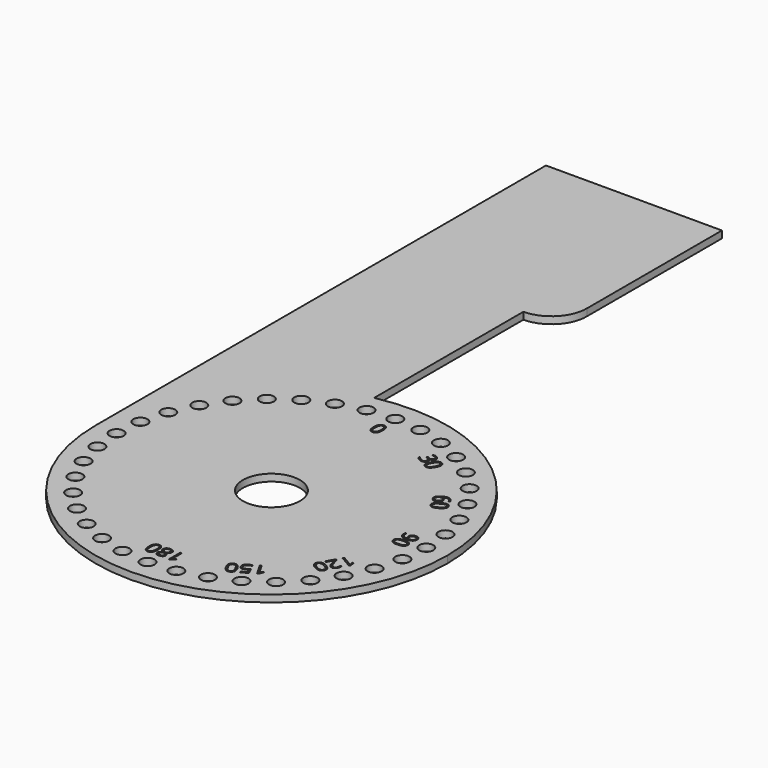
from build123d import *

# Parameters (mm, degrees)
F1_DEPTH     = 1
F3_D         = 2
F4_TEXT_SIZE = 2.7777777778
F5_DEPTH     = 1
F6_TEXT_SIZE = 2.7777777778
F7_DEPTH     = 25
F8_TEXT_SIZE = 2.7777777778
F9_DEPTH     = 25
F11_DEPTH    = 1


# Not quite as in the source:
# - a feature names something its author has since deleted; it is built from what else it names
# - Text() gives the source's letters only with a copy of the font that has no kerning and outlines rounded to 1/6400 em; it was checked with that copy


with BuildPart() as f1:
    # F0 (on Top) → F1 (new body)
    with BuildSketch(Plane.XY):
        with BuildLine():
            ThreePointArc((-25, 0), (0, 25), (25, 0))
            Line((25, 0), (25, 35))
            Line((25, 35), (0, 60))
            Line((0, 60), (0, 65))
            Line((0, 65), (25, 65))
            Line((25, 65), (25, 80))
            Line((25, 80), (-25, 80))
            Line((-25, 80), (-25, 0))
        make_face()
        with BuildLine():
            Line((25, 0), (4.05, 0))
            ThreePointArc((4.05, 0), (0, -4.05), (-4.05, 0))
            Line((-4.05, 0), (-25, 0))
            ThreePointArc((-25, 0), (0, -25), (25, 0))
        make_face()
        with BuildLine():
            ThreePointArc((-4.05, 0), (0, 4.05), (4.05, 0))
            Line((4.05, 0), (25, 0))
            ThreePointArc((25, 0), (0, 25), (-25, 0))
            Line((-25, 0), (-4.05, 0))
        make_face()
        Polygon((0, 60), (25, 35), (25, 65), (0, 65), align=None)
    extrude(amount=-F1_DEPTH)

    # F3 (through all)
    with Locations(Plane.XY):
        with Locations((0, -22), (0, 0), (7.5244431532, -20.6732376573), (3.8202599087, -21.6657705663), (-22, 0), (21.6657705663, -3.8202599087), (-21.6657705663, -3.8202599087), (19.0525588833, -11), (-16.8529777486, 14.1413274131), (-21.6657705663, 3.8202599087), (16.8529777486, 14.1413274131), (-7.5244431532, -20.6732376573), (-7.5244431532, 20.6732376573), (-14.1413274131, 16.8529777486), (22, 0), (-14.1413274131, -16.8529777486), (-20.6732376573, 7.5244431532), (-16.8529777486, -14.1413274131), (14.1413274131, -16.8529777486), (11, 19.0525588833), (-19.0525588833, 11), (-20.6732376573, -7.5244431532), (20.6732376573, -7.5244431532), (3.8202599087, 21.6657705663), (0, 22), (-11, -19.0525588833), (21.6657705663, 3.8202599087), (14.1413274131, 16.8529777486), (-11, 19.0525588833), (7.5244431532, 20.6732376573), (11, -19.0525588833), (-3.8202599087, 21.6657705663), (20.6732376573, 7.5244431532), (19.0525588833, 11), (-3.8202599087, -21.6657705663), (16.8529777486, -14.1413274131), (-19.0525588833, -11)):
            Hole(F3_D / 2)

    # F4 (on face) → F5 (cut, through all)
    with BuildSketch(Plane.XY):
        with Locations((-0.8151041667, 18)):
            Text('0', F4_TEXT_SIZE, font='Open Sans', text_align=(TextAlign.LEFT, TextAlign.BOTTOM))
    extrude(amount=-F5_DEPTH, mode=Mode.SUBTRACT)

    # F6 (on face) → F7 (cut)
    with BuildSketch(Plane.XY):
        with Locations(Location((7.6064283053, 16.3930362612), (0, 0, -30))):
            Text('30', F6_TEXT_SIZE, font='Open Sans', text_align=(TextAlign.LEFT, TextAlign.BOTTOM))
        with Locations(Location((18, 1.6091579861), (0, 0, -90))):
            Text('90', F6_TEXT_SIZE, font='Open Sans', text_align=(TextAlign.LEFT, TextAlign.BOTTOM))
        with Locations(Location((14.7838782751, 10.3935716947), (0, 0, -60))):
            Text('60', F6_TEXT_SIZE, font='Open Sans', text_align=(TextAlign.LEFT, TextAlign.BOTTOM))
    extrude(amount=-F7_DEPTH, mode=Mode.SUBTRACT)

    # F8 (on face) → F9 (cut)
    with BuildSketch(Plane.XY):
        with Locations(Location((11.0812424743, -14.3868513653), (0, 0, -150))):
            Text('150', F8_TEXT_SIZE, font='Open Sans', text_align=(TextAlign.LEFT, TextAlign.BOTTOM))
        with Locations(Location((2.4032118056, -18), (0, 0, 180))):
            Text('180', F8_TEXT_SIZE, font='Open Sans', text_align=(TextAlign.LEFT, TextAlign.BOTTOM))
        with Locations(Location((16.7900631709, -6.9187575257), (0, 0, -120))):
            Text('120', F8_TEXT_SIZE, font='Open Sans', text_align=(TextAlign.LEFT, TextAlign.BOTTOM))
        with Locations((175.0965838585, 43.4660910182)):
            Text('120', F8_TEXT_SIZE, font='Open Sans', text_align=(TextAlign.LEFT, TextAlign.BOTTOM))
    extrude(amount=-F9_DEPTH, mode=Mode.SUBTRACT)

    # F10 (on face) → F11 (cut, through all)
    with BuildSketch(Plane.XY):
        with BuildLine():
            ThreePointArc((-5, 24.4948974278), (15.8113883008, 19.364916731), (25, 0))
            Line((25, 0), (25, 80))
            Line((25, 80), (0, 80))
            Line((0, 80), (0, 56))
            ThreePointArc((0, 56), (-1.4644660941, 52.4644660941), (-5, 51))
            Line((-5, 51), (-5, 24.4948974278))
        make_face()
    extrude(amount=-F11_DEPTH, mode=Mode.SUBTRACT)


solid = f1.part
